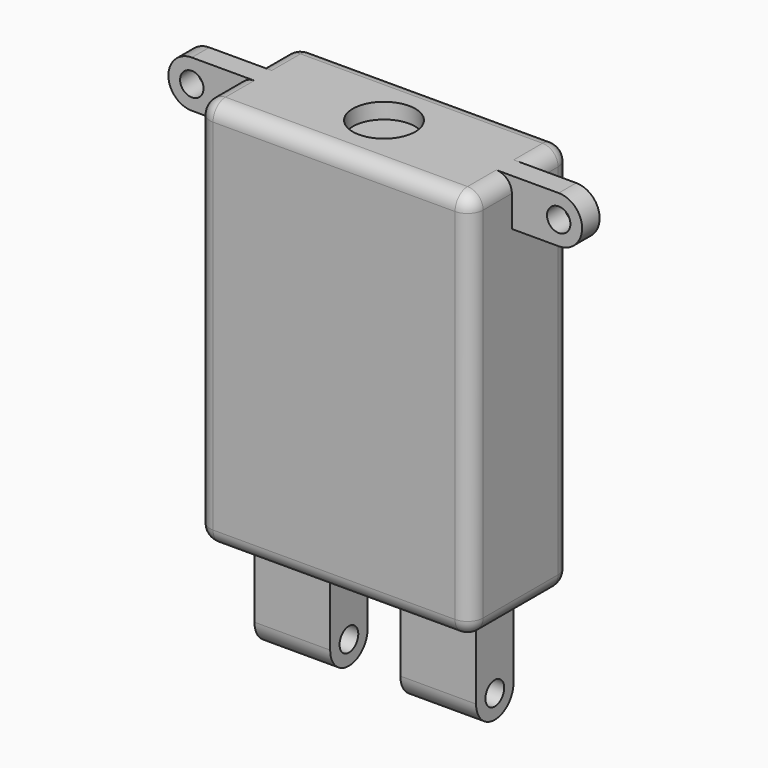
from build123d import *

# Parameters (mm, degrees)
F1_DEPTH      = 17.5
F2_W          = 6.3770967536
F2_H          = 17.8738087416
F2_W_2        = 4.4888177946
F3_DEPTH      = 12.5
F5_R          = 4
F6_DEPTH      = 2
F7_R          = 1.5
F8_DEPTH      = 1.4
F10_R         = 2
F11_T1_DEPTH  = 12
F11_T3_DEPTH  = 4.6
F11_T5_DEPTH  = 4.6
F11_S9_W      = 2
F11_S9_H      = 2
F11_T10_DEPTH = 2
F11_S15_W     = 2
F11_S15_H     = 2
F11_T16_DEPTH = 2
F11_S21_W     = 2
F11_S21_H     = 2
F11_T22_DEPTH = 2
F11_S27_W     = 2
F11_S27_H     = 2
F11_T28_DEPTH = 2
F11_S33_W     = 2
F11_S33_H     = 2
F11_T34_DEPTH = 2
F11_S39_W     = 2
F11_S39_H     = 2
F11_T40_DEPTH = 2
F11_S45_W     = 2
F11_S45_H     = 2
F11_T46_DEPTH = 2
F11_S51_W     = 2
F11_S51_H     = 2
F11_T52_DEPTH = 2
F11_T58_DEPTH = 9.6
F11_T63_DEPTH = 9.6
F11_T68_DEPTH = 9.6
F11_T73_DEPTH = 9.6


# Not quite as in the source:
# - a fillet or chamfer that OpenCascade refuses, or shapes differently, is made with other operations: its cross-section is extruded or revolved along the edge and cut away or added


with BuildPart() as f1:
    # F0 (on Right) → F1 (new body, symmetric)
    with BuildSketch(Plane.YZ):
        Polygon((3, 0), (8, 0), (8, 50), (-8, 50), (-8, 0), (-3, 0), align=None)
        with BuildLine():
            Line((3, -10), (3, 0))
            Line((3, 0), (-3, 0))
            Line((-3, 0), (-3, -10))
            ThreePointArc((-3, -10), (0, -7), (3, -10))
        make_face()
        with BuildLine():
            ThreePointArc((-3, -10), (0, -13), (3, -10))
            ThreePointArc((3, -10), (0, -7), (-3, -10))
        make_face()
        with BuildLine():
            ThreePointArc((1.5, -10), (0, -11.5), (-1.5, -10))
            ThreePointArc((-1.5, -10), (0, -8.5), (1.5, -10))
        make_face(mode=Mode.SUBTRACT)
    extrude(amount=F1_DEPTH, both=True)

    # F2 (on Front) → F3 (cut, symmetric)
    with BuildSketch(Plane.XZ):
        with Locations((-17.3829572741, -8.9369043708)):
            Rectangle(F2_W, F2_H)
        Polygon((-0.0055911027, 0), (-4.4944088973, 0), (-4.4944088973, -17.8738087416), (-0.0055911027, -17.8738087416), (0.0055911027, -17.8738087416), (0.0055911027, 0), align=None)
        with Locations((2.25, -8.9369043708)):
            Rectangle(F2_W_2, F2_H)
        with Locations((17.3829572741, -8.9369043708)):
            Rectangle(F2_W, F2_H)
    extrude(amount=F3_DEPTH, both=True, mode=Mode.SUBTRACT)

    # F5 (on offset) → F6 (cut)
    with BuildSketch(Plane.XY.offset(50)):
        Circle(F5_R)
    extrude(amount=-F6_DEPTH, mode=Mode.SUBTRACT)

    # F7 (on Front) → F8 (join, symmetric)
    with BuildSketch(Plane.XZ):
        with BuildLine():
            Line((23.5, 50), (17.5, 50))
            Line((17.5, 50), (17.5, 44))
            Line((17.5, 44), (23.5, 44))
            ThreePointArc((23.5, 44), (26.5, 47), (23.5, 50))
        make_face()
        with Locations((23.5, 47)):
            Circle(F7_R, mode=Mode.SUBTRACT)
    extrude(amount=F8_DEPTH, both=True)

    # F9: F1 across plane


with BuildPart() as f1_1:
    add(f1.part)
    add(f1.part.mirror(Plane.YZ))

    # F10
    f10_edges = [f1_1.edges().sort_by_distance(p)[0] for p in [
        (0, -8, 50),
        (-17.5, -8, 25),
        (0, -8, 0),
        (17.5, -8, 25),
        (0, 8, 0),
        (-17.5, 8, 25),
        (0, 8, 50),
        (17.5, 8, 25),
    ]]
    fillet(f10_edges, radius=F10_R)

    # F11: fillet of radius 2 on 8 edges, made by hand

    # F11_s2 → F11_t1 (cut)
    with BuildSketch(Plane.XZ.offset(-6)):
        with BuildLine():
            ThreePointArc((15.5, 0), (16.9142135624, 0.5857864376), (17.5, 2))
            Line((17.5, 2), (17.5, 0))
            Line((17.5, 0), (15.5, 0))
        make_face()
        with BuildLine():
            ThreePointArc((-15.5, 0), (-16.9142135624, 0.5857864376), (-17.5, 2))
            Line((-17.5, 2), (-17.5, 0))
            Line((-17.5, 0), (-15.5, 0))
        make_face()
    extrude(amount=F11_T1_DEPTH, mode=Mode.SUBTRACT)

    # F11_s4 → F11_t3 (cut)
    with BuildSketch(Plane.XZ.offset(-6)):
        with BuildLine():
            ThreePointArc((17.5, 48), (16.9142135624, 49.4142135624), (15.5, 50))
            Line((15.5, 50), (17.5, 50))
            Line((17.5, 50), (17.5, 48))
        make_face()
        with BuildLine():
            ThreePointArc((-17.5, 48), (-16.9142135624, 49.4142135624), (-15.5, 50))
            Line((-15.5, 50), (-17.5, 50))
            Line((-17.5, 50), (-17.5, 48))
        make_face()
    extrude(amount=F11_T3_DEPTH, mode=Mode.SUBTRACT)

    # F11_s6 → F11_t5 (cut)
    with BuildSketch(Plane.XZ.offset(1.4)):
        with BuildLine():
            ThreePointArc((17.5, 48), (16.9142135624, 49.4142135624), (15.5, 50))
            Line((15.5, 50), (17.5, 50))
            Line((17.5, 50), (17.5, 48))
        make_face()
        with BuildLine():
            ThreePointArc((-17.5, 48), (-16.9142135624, 49.4142135624), (-15.5, 50))
            Line((-15.5, 50), (-17.5, 50))
            Line((-17.5, 50), (-17.5, 48))
        make_face()
    extrude(amount=F11_T5_DEPTH, mode=Mode.SUBTRACT)


with BuildPart() as f11_tool8:
    # F11_s9 → F11_t10 (new body)
    with BuildSketch(Plane.YZ.offset(-15.5)):
        with Locations((7, 49)):
            Rectangle(F11_S9_W, F11_S9_H)
    extrude(amount=-F11_T10_DEPTH)

    # F11_s11 → F11_t12 (revolve, cut)
    with BuildSketch(Plane(origin=(-15.5, 6, 48), x_dir=(0, -0.7071067812, -0.7071067812), z_dir=(0, 0.7071067812, -0.7071067812))):
        with BuildLine():
            ThreePointArc((0, -2), (2, 0), (0, 2))
            Line((0, 2), (0, -2))
        make_face()
    revolve(axis=Axis((-15.5, 6, 48), (-1, 0, 0)), mode=Mode.SUBTRACT)


with BuildPart() as f1_2:
    add(f1_1.part)

    # F11_t7: cut F11_tool8
    add(f11_tool8.part, mode=Mode.SUBTRACT)


with BuildPart() as f11_tool14:
    # F11_s15 → F11_t16 (new body)
    with BuildSketch(Plane.YZ.offset(-15.5)):
        with Locations((-7, 49)):
            Rectangle(F11_S15_W, F11_S15_H)
    extrude(amount=-F11_T16_DEPTH)

    # F11_s17 → F11_t18 (revolve, cut)
    with BuildSketch(Plane(origin=(-15.5, -6, 48), x_dir=(0, 0.7071067812, -0.7071067812), z_dir=(0, 0.7071067812, 0.7071067812))):
        with BuildLine():
            ThreePointArc((0, -2), (2, 0), (0, 2))
            Line((0, 2), (0, -2))
        make_face()
    revolve(axis=Axis((-15.5, -6, 48), (-1, 0, 0)), mode=Mode.SUBTRACT)


with BuildPart() as f1_3:
    add(f1_2.part)

    # F11_t13: cut F11_tool14
    add(f11_tool14.part, mode=Mode.SUBTRACT)


with BuildPart() as f11_tool20:
    # F11_s21 → F11_t22 (new body)
    with BuildSketch(Plane.YZ.offset(15.5)):
        with Locations((-7, 49)):
            Rectangle(F11_S21_W, F11_S21_H)
    extrude(amount=F11_T22_DEPTH)

    # F11_s23 → F11_t24 (revolve, cut)
    with BuildSketch(Plane(origin=(15.5, -6, 48), x_dir=(0, 0.7071067812, -0.7071067812), z_dir=(0, -0.7071067812, -0.7071067812))):
        with BuildLine():
            ThreePointArc((0, -2), (2, 0), (0, 2))
            Line((0, 2), (0, -2))
        make_face()
    revolve(axis=Axis((15.5, -6, 48), (1, 0, 0)), mode=Mode.SUBTRACT)


with BuildPart() as f1_4:
    add(f1_3.part)

    # F11_t19: cut F11_tool20
    add(f11_tool20.part, mode=Mode.SUBTRACT)


with BuildPart() as f11_tool26:
    # F11_s27 → F11_t28 (new body)
    with BuildSketch(Plane.YZ.offset(15.5)):
        with Locations((7, 49)):
            Rectangle(F11_S27_W, F11_S27_H)
    extrude(amount=F11_T28_DEPTH)

    # F11_s29 → F11_t30 (revolve, cut)
    with BuildSketch(Plane(origin=(15.5, 6, 48), x_dir=(0, -0.7071067812, -0.7071067812), z_dir=(0, -0.7071067812, 0.7071067812))):
        with BuildLine():
            ThreePointArc((0, -2), (2, 0), (0, 2))
            Line((0, 2), (0, -2))
        make_face()
    revolve(axis=Axis((15.5, 6, 48), (1, 0, 0)), mode=Mode.SUBTRACT)


with BuildPart() as f1_5:
    add(f1_4.part)

    # F11_t25: cut F11_tool26
    add(f11_tool26.part, mode=Mode.SUBTRACT)


with BuildPart() as f11_tool32:
    # F11_s33 → F11_t34 (new body)
    with BuildSketch(Plane.XY.offset(2)):
        with Locations((-16.5, -7)):
            Rectangle(F11_S33_W, F11_S33_H)
    extrude(amount=-F11_T34_DEPTH)

    # F11_s35 → F11_t36 (revolve, cut)
    with BuildSketch(Plane(origin=(-15.5, -6, 2), x_dir=(0.7071067812, 0.7071067812, 0), z_dir=(-0.7071067812, 0.7071067812, 0))):
        with BuildLine():
            ThreePointArc((0, -2), (2, 0), (0, 2))
            Line((0, 2), (0, -2))
        make_face()
    revolve(axis=Axis((-15.5, -6, 2), (0, 0, -1)), mode=Mode.SUBTRACT)


with BuildPart() as f1_6:
    add(f1_5.part)

    # F11_t31: cut F11_tool32
    add(f11_tool32.part, mode=Mode.SUBTRACT)


with BuildPart() as f11_tool38:
    # F11_s39 → F11_t40 (new body)
    with BuildSketch(Plane.XY.offset(2)):
        with Locations((-16.5, 7)):
            Rectangle(F11_S39_W, F11_S39_H)
    extrude(amount=-F11_T40_DEPTH)

    # F11_s41 → F11_t42 (revolve, cut)
    with BuildSketch(Plane(origin=(-15.5, 6, 2), x_dir=(0.7071067812, -0.7071067812, 0), z_dir=(0.7071067812, 0.7071067812, 0))):
        with BuildLine():
            ThreePointArc((0, -2), (2, 0), (0, 2))
            Line((0, 2), (0, -2))
        make_face()
    revolve(axis=Axis((-15.5, 6, 2), (0, 0, -1)), mode=Mode.SUBTRACT)


with BuildPart() as f1_7:
    add(f1_6.part)

    # F11_t37: cut F11_tool38
    add(f11_tool38.part, mode=Mode.SUBTRACT)


with BuildPart() as f11_tool44:
    # F11_s45 → F11_t46 (new body)
    with BuildSketch(Plane.XY.offset(2)):
        with Locations((16.5, 7)):
            Rectangle(F11_S45_W, F11_S45_H)
    extrude(amount=-F11_T46_DEPTH)

    # F11_s47 → F11_t48 (revolve, cut)
    with BuildSketch(Plane(origin=(15.5, 6, 2), x_dir=(-0.7071067812, -0.7071067812, 0), z_dir=(0.7071067812, -0.7071067812, 0))):
        with BuildLine():
            ThreePointArc((0, -2), (2, 0), (0, 2))
            Line((0, 2), (0, -2))
        make_face()
    revolve(axis=Axis((15.5, 6, 2), (0, 0, -1)), mode=Mode.SUBTRACT)


with BuildPart() as f1_8:
    add(f1_7.part)

    # F11_t43: cut F11_tool44
    add(f11_tool44.part, mode=Mode.SUBTRACT)


with BuildPart() as f11_tool50:
    # F11_s51 → F11_t52 (new body)
    with BuildSketch(Plane.XY.offset(2)):
        with Locations((16.5, -7)):
            Rectangle(F11_S51_W, F11_S51_H)
    extrude(amount=-F11_T52_DEPTH)

    # F11_s53 → F11_t54 (revolve, cut)
    with BuildSketch(Plane(origin=(15.5, -6, 2), x_dir=(-0.7071067812, 0.7071067812, 0), z_dir=(-0.7071067812, -0.7071067812, 0))):
        with BuildLine():
            ThreePointArc((0, -2), (2, 0), (0, 2))
            Line((0, 2), (0, -2))
        make_face()
    revolve(axis=Axis((15.5, -6, 2), (0, 0, -1)), mode=Mode.SUBTRACT)


with BuildPart() as f1_9:
    add(f1_8.part)

    # F11_t49: cut F11_tool50
    add(f11_tool50.part, mode=Mode.SUBTRACT)


with BuildPart() as f11_tool56:
    # F11_s57 → F11_t58 (new body)
    with BuildSketch(Plane.XZ.offset(-6)):
        with BuildLine():
            ThreePointArc((17.5, 48), (16.9142135624, 49.4142135624), (15.5, 50))
            Line((15.5, 50), (17.5, 50))
            Line((17.5, 50), (17.5, 48))
        make_face()
    extrude(amount=F11_T58_DEPTH)

    split(bisect_by=Plane.XZ.offset(1.4), keep=Keep.TOP)


with BuildPart() as f1_10:
    add(f1_9.part)

    # F11_t55: cut F11_tool56
    add(f11_tool56.part, mode=Mode.SUBTRACT)


with BuildPart() as f11_tool61:
    # F11_s62 → F11_t63 (new body)
    with BuildSketch(Plane.XZ.offset(-3.6)):
        with BuildLine():
            ThreePointArc((17.5, 48), (16.9142135624, 49.4142135624), (15.5, 50))
            Line((15.5, 50), (17.5, 50))
            Line((17.5, 50), (17.5, 48))
        make_face()
    extrude(amount=F11_T63_DEPTH)

    split(bisect_by=Plane.XZ.offset(-1.4), keep=Keep.BOTTOM)


with BuildPart() as f1_11:
    add(f1_10.part)

    # F11_t60: cut F11_tool61
    add(f11_tool61.part, mode=Mode.SUBTRACT)


with BuildPart() as f11_tool66:
    # F11_s67 → F11_t68 (new body)
    with BuildSketch(Plane.XZ.offset(-3.6)):
        with BuildLine():
            ThreePointArc((-17.5, 48), (-16.9142135624, 49.4142135624), (-15.5, 50))
            Line((-15.5, 50), (-17.5, 50))
            Line((-17.5, 50), (-17.5, 48))
        make_face()
    extrude(amount=F11_T68_DEPTH)

    split(bisect_by=Plane.XZ.offset(-1.4), keep=Keep.BOTTOM)


with BuildPart() as f1_12:
    add(f1_11.part)

    # F11_t65: cut F11_tool66
    add(f11_tool66.part, mode=Mode.SUBTRACT)


with BuildPart() as f11_tool71:
    # F11_s72 → F11_t73 (new body)
    with BuildSketch(Plane.XZ.offset(-6)):
        with BuildLine():
            ThreePointArc((-17.5, 48), (-16.9142135624, 49.4142135624), (-15.5, 50))
            Line((-15.5, 50), (-17.5, 50))
            Line((-17.5, 50), (-17.5, 48))
        make_face()
    extrude(amount=F11_T73_DEPTH)

    split(bisect_by=Plane.XZ.offset(1.4), keep=Keep.TOP)


with BuildPart() as f1_13:
    add(f1_12.part)

    # F11_t70: cut F11_tool71
    add(f11_tool71.part, mode=Mode.SUBTRACT)


solid = f1_13.part
